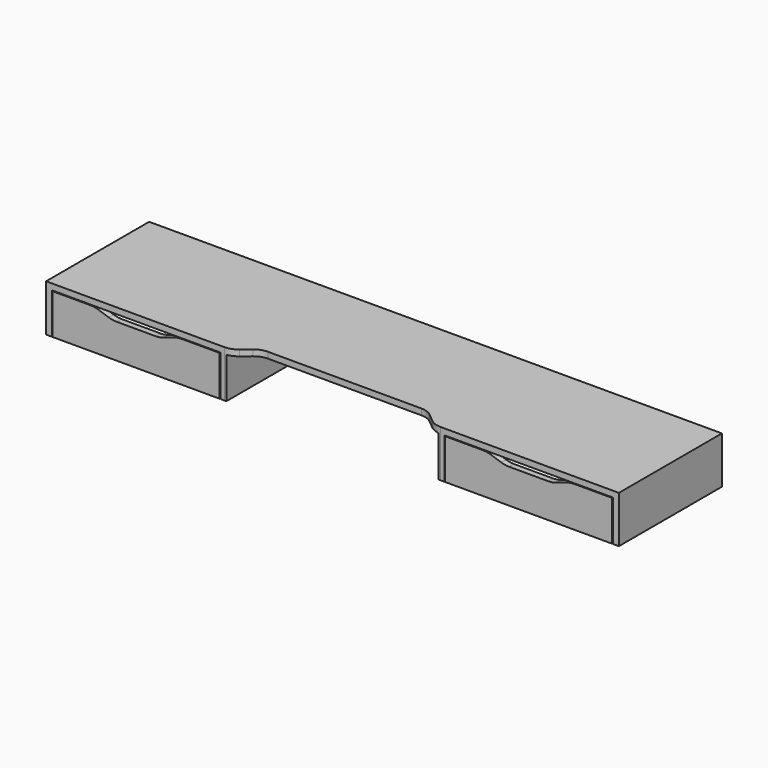
from build123d import *

# Parameters (mm, degrees)
F0_W      = 1200.15
F0_H      = 269.875
F1_DEPTH  = 12.7
F2_W      = 269.875
F2_H      = 85.725
F3_DEPTH  = 12.7
F4_W      = 269.875
F4_H      = 85.725
F5_DEPTH  = 12.7
F6_W      = 12.7
F6_H      = 269.875
F7_DEPTH  = 85.725
F9_DEPTH  = 12.7
F10_R     = 38.1
F11_W     = 349.885
F11_H     = 84.455
F12_DEPTH = 12.7
F13_W     = 349.885
F13_H     = 84.455
F14_DEPTH = 12.7
F16_DEPTH = 12.7
F17_R     = 50.8
F19_DEPTH = 12.7
F20_R     = 50.8


with BuildPart() as f1:
    # F0 (on Top) → F1 (new body)
    with BuildSketch(Plane.XY):
        Rectangle(F0_W, F0_H)
    extrude(amount=F1_DEPTH)

    # F2 (on face) → F3 (join)
    with BuildSketch(Plane(origin=(-600.075, 0, 0), x_dir=(0, -1, 0), z_dir=(-1, 0, 0))):
        with Locations((0, -42.8625)):
            Rectangle(F2_W, F2_H)
    extrude(amount=-F3_DEPTH)

    # F4 (on face) → F5 (join)
    with BuildSketch(Plane.YZ.offset(600.075)):
        with Locations((0, -42.8625)):
            Rectangle(F4_W, F4_H)
    extrude(amount=-F5_DEPTH)

    # F6 (on face) → F7 (join)
    with BuildSketch(Plane(origin=(0, 0, 0), x_dir=(1, 0, 0), z_dir=(0, 0, -1))):
        with Locations((228.6, 0)):
            Rectangle(F6_W, F6_H)
        with Locations((-228.6, 0)):
            Rectangle(F6_W, F6_H)
    extrude(amount=F7_DEPTH)

    # F8 (on face) → F9 (cut)
    with BuildSketch(Plane.XY.offset(12.7)):
        Polygon((174.625, -103.1875), (-174.625, -103.1875), (-212.725, -134.9375), (212.725, -134.9375), align=None)
    extrude(amount=-F9_DEPTH, mode=Mode.SUBTRACT)

    # F10
    f10_edges = [f1.edges().sort_by_distance(p)[0] for p in [
        (-174.625, -103.1875, 6.35),
        (-212.725, -134.9375, 6.35),
        (174.625, -103.1875, 6.35),
        (212.725, -134.9375, 6.35),
    ]]
    fillet(f10_edges, radius=F10_R)


with BuildPart() as f12:
    # F11 (on face) → F12 (new body)
    with BuildSketch(Plane.XZ.offset(134.9375)):
        with Locations((-411.1625, -43.4975)):
            Rectangle(F11_W, F11_H)
    extrude(amount=-F12_DEPTH)

    # F15 (on face) → F16 (cut)
    with BuildSketch(Plane.XZ.offset(134.9375)):
        Polygon((-323.69125, -1.27), (-498.63375, -1.27), (-460.53375, -13.97), (-361.79125, -13.97), align=None)
    extrude(amount=-F16_DEPTH, mode=Mode.SUBTRACT)

    # F17
    f17_edges = [f12.edges().sort_by_distance(p)[0] for p in [
        (-498.63375, -128.5875, -1.27),
        (-460.53375, -128.5875, -13.97),
        (-361.79125, -128.5875, -13.97),
        (-323.69125, -128.5875, -1.27),
    ]]
    fillet(f17_edges, radius=F17_R)


with BuildPart() as f14:
    # F13 (on face) → F14 (new body)
    with BuildSketch(Plane.XZ.offset(134.9375)):
        with Locations((411.1625, -43.4975)):
            Rectangle(F13_W, F13_H)
    extrude(amount=-F14_DEPTH)

    # F18 (on face) → F19 (cut)
    with BuildSketch(Plane.XZ.offset(134.9375)):
        Polygon((498.63375, -1.27), (323.69125, -1.27), (361.79125, -13.97), (460.53375, -13.97), align=None)
    extrude(amount=-F19_DEPTH, mode=Mode.SUBTRACT)

    # F20
    f20_edges = [f14.edges().sort_by_distance(p)[0] for p in [
        (323.69125, -128.5875, -1.27),
        (361.79125, -128.5875, -13.97),
        (460.53375, -128.5875, -13.97),
        (498.63375, -128.5875, -1.27),
    ]]
    fillet(f20_edges, radius=F20_R)


solid = Compound([f1.part, f12.part, f14.part])
